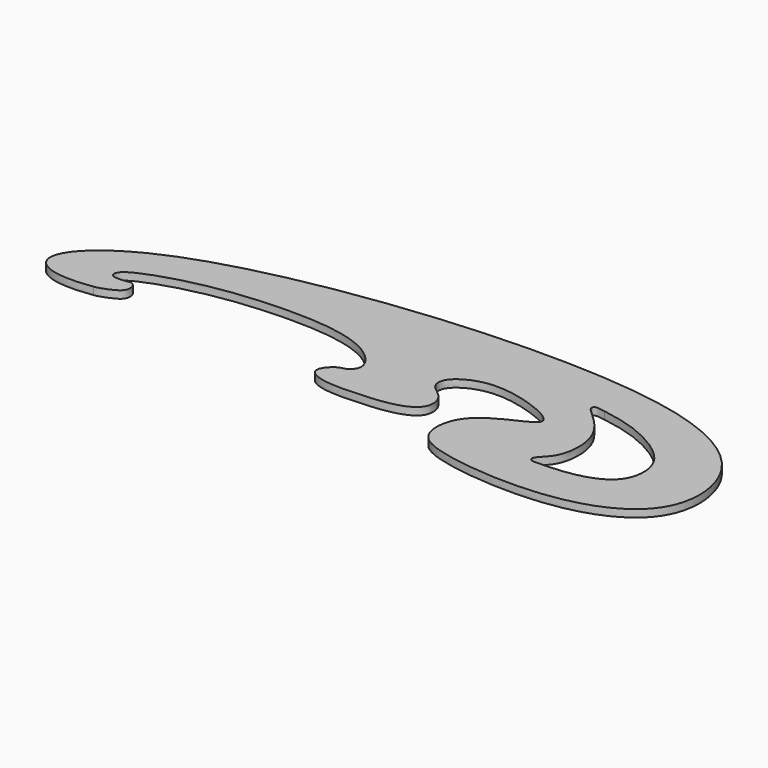
from build123d import *

# Parameters (mm, degrees)
F1_DEPTH = 1.6002


with BuildPart() as f1:
    # F0 (on Top) → F1 (new body)
    with BuildSketch(Plane.XY):
        with BuildLine():
            add(Edge.make_bspline(
                [(-59.4281516969, -11.7521779612), (-66.9164822654, -12.8709442898), (-76.3164245519, -9.429170469), (-56.1853390615, 12.1290322868), (37.2411499356, 21.3747454249), (67.1846066296, 4.2762865141), (67.8776118258, -16.2495153326), (49.751326097, -25.0750892546), (25.8428346418, -23.4780914994), (16.3790808941, -19.5256792252), (17.5051118184, -9.5076657662), (23.6086996224, -6.6401017182), (27.0235463977, -5.0351535901)],
                knots=[0, 0, 0, 0, 0.078614784, 0.1761620845, 0.3922097147, 0.5152319577, 0.6007533714, 0.6945613856, 0.8037814335, 0.8684801047, 0.9291583522, 1, 1, 1, 1], degree=3))
            add(Edge.make_bspline(
                [(27.0235463977, -5.0351535901), (27.9190652072, -4.5834821649), (32.4908252274, -2.5560546758), (20.8155394335, 2.3350301627), (12.2711486614, 2.4745694206), (6.9656354837, -1.1716664139), (7.4989671528, -4.6884361599), (10.9036388063, -6.3022749874), (12.0269407688, -10.4784588795), (8.4312903078, -13.7857399523), (-1.0235506006, -14.6483731557), (-9.0125217752, -14.6373863221), (-12.3999965927, -12.0736636247), (-9.437447283, -8.7404377808), (-7.683696338, -8.8834853849), (-5.4457223037, -6.5984425977), (-8.2550843828, -2.159880639), (-15.8952158838, 1.4873574473), (-30.2180479926, 2.2400053595), (-45.630038844, 0.6207922898), (-56.467058748, -2.880221801), (-59.6054892668, -4.9650623241), (-59.6844776543, -6.522343106), (-58.5715366776, -6.9914043396), (-56.3993310894, -6.8516598969), (-55.2040604805, -6.4873125944), (-54.1202164401, -7.5942851869), (-54.219163665, -9.5280252235), (-56.0786600075, -10.739242353), (-58.3472400904, -11.5997940302), (-59.4281516969, -11.7521779612)],
                knots=[0, 0, 0, 0, 0.0316762124, 0.0835129808, 0.136786603, 0.1764819497, 0.2045564521, 0.2367163129, 0.2690869933, 0.3034836259, 0.3566867001, 0.4058817584, 0.4351001107, 0.466717322, 0.4894264735, 0.5157835738, 0.5511499619, 0.6001977553, 0.6650574577, 0.7341508119, 0.79147957, 0.822282137, 0.8402649593, 0.8575340845, 0.8829436918, 0.901513176, 0.9208863461, 0.9429867155, 0.967826206, 1, 1, 1, 1], degree=3))
        make_face()
        with BuildLine():
            add(Edge.make_bspline(
                [(37.4975651503, -15.2385588735), (37.1680743992, -15.238462016), (36.0277063648, -14.1324504181), (40.3966497501, -11.4893054509), (40.8387537404, -1.5514900565), (34.9825153997, 3.9730101163), (32.9464545412, 5.7143896423), (33.2652279241, 6.8919251835), (34.7428570913, 6.5470457525), (35.6364026666, 6.3988603652)],
                knots=[0, 0, 0, 0, 0.0811345183, 0.237069927, 0.4759051405, 0.6972164307, 0.8170806333, 0.8813630931, 1, 1, 1, 1], degree=3))
            add(Edge.make_bspline(
                [(35.6364026666, 6.3988603652), (41.2198901176, 5.5845491588), (48.8143220843, 2.5650641532), (55.0926931084, -3.5409120106), (54.2497298479, -12.1575681334), (45.4932475752, -15.1515383272), (40.1554287042, -15.2107121917), (37.4975651503, -15.2385588735)],
                knots=[0, 0, 0, 0, 0.2514977472, 0.4390920088, 0.6156329214, 0.808452436, 1, 1, 1, 1], degree=3))
        make_face(mode=Mode.SUBTRACT)
    extrude(amount=F1_DEPTH)


solid = f1.part
